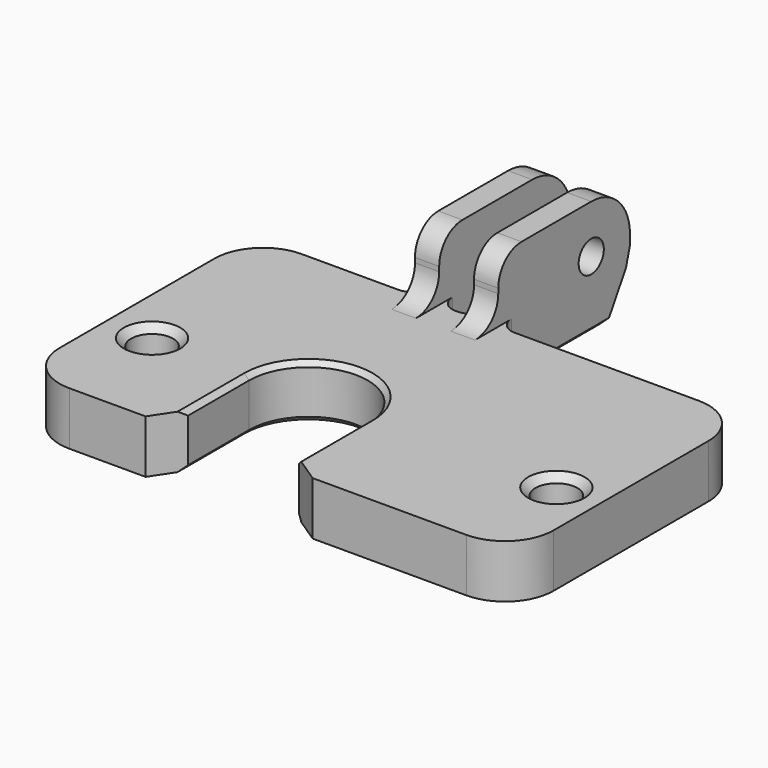
from build123d import *

# Parameters (mm, degrees)
F0_R          = 2.1666665
F1_DEPTH      = 5.5
F2_SIZE       = 0.75
F3_W          = 51
F3_H          = 8
F4_DEPTH      = 5.5
F5_SIZE       = 0.5
F6_W          = 2.5
F6_H          = 17
F7_DEPTH      = 12
F8_R          = 1.625
F9_DEPTH      = 25.301
F10_T1_DEPTH  = 2.5
F10_T3_DEPTH  = 2.5
F10_T8_DEPTH  = 17.5
F10_T14_DEPTH = 17.5
F10_T17_DEPTH = 17.5
F10_T19_DEPTH = 17.5
F11_R         = 5
F12_SIZE2     = 3
F12_SIZE      = 5
F12_2_SIZE2   = 3
F12_2_SIZE    = 5
F13_SIZE      = 1
F14_R         = 5
F15_SIZE2     = 2
F15_SIZE      = 3
F15_2_SIZE2   = 2
F15_2_SIZE    = 3
F16_T1_DEPTH  = 15.285841494
F16_T3_DEPTH  = 4.0033035506
F16_T5_DEPTH  = 4.0033035506
F17_R         = 1.7


# Not quite as in the source:
# - a fillet or chamfer that OpenCascade refuses, or shapes differently, is made with other operations: its cross-section is extruded or revolved along the edge and cut away or added


with BuildPart() as f1:
    # F0 (on Top) → F1 (new body)
    with BuildSketch(Plane.XY):
        with BuildLine():
            Line((25.5, 11), (-25.5, 11))
            Line((-25.5, 11), (-25.5, -11))
            Line((-25.5, -11), (-10.625, -11))
            Line((-10.625, -11), (-10.625, -0.125))
            ThreePointArc((-10.625, -0.125), (-4.5, 6), (1.625, -0.125))
            Line((1.625, -0.125), (1.625, -11))
            Line((1.625, -11), (25.5, -11))
            Line((25.5, -11), (25.5, 11))
        make_face()
        with Locations((-20.75, 0)):
            Circle(F0_R, mode=Mode.SUBTRACT)
        with Locations((21, 0)):
            Circle(F0_R, mode=Mode.SUBTRACT)
    extrude(amount=F1_DEPTH)

    # F2
    f2_edges = [f1.edges().sort_by_distance(p)[0] for p in [
        (-22.916666, 0, 0),
        (18.833334, 0, 0),
        (18.833334, 0, 5.5),
        (-22.916666, 0, 5.5),
    ]]
    chamfer(f2_edges, length=F2_SIZE)

    # F3 (on Top) → F4 (join, through all)
    with BuildSketch(Plane.XY):
        with Locations((0, 15)):
            Rectangle(F3_W, F3_H)
    extrude(amount=F4_DEPTH)

    # F5
    f5_edges = [f1.edges().sort_by_distance(p)[0] for p in [
        (-4.5, 6, 5.5),
        (-4.5, 6, 0),
        (-10.625, -5.5625, 5.5),
        (-10.625, -5.5625, 0),
        (1.625, -5.5625, 0),
        (1.625, -5.5625, 5.5),
    ]]
    chamfer(f5_edges, length=F5_SIZE)

    # F6 (on Top) → F7 (join)
    with BuildSketch(Plane.XY):
        with Locations((-7.55, 27.5)):
            Rectangle(F6_W, F6_H)
        with Locations((-1.45, 27.5)):
            Rectangle(F6_W, F6_H)
    extrude(amount=F7_DEPTH)

    # F8 (on face) → F9 (cut, through all)
    with BuildSketch(Plane.YZ.offset(-0.2)):
        with Locations((31, 7)):
            Circle(F8_R)
    extrude(amount=-F9_DEPTH, mode=Mode.SUBTRACT)

    # F10: fillet of radius 3 on 5 edges, made by hand

    # F10_s2 → F10_t1 (join)
    with BuildSketch(Plane.YZ.offset(-2.7)):
        with BuildLine():
            ThreePointArc((16, 5.5), (18.1213203436, 6.3786796564), (19, 8.5))
            Line((19, 8.5), (19, 5.5))
            Line((19, 5.5), (16, 5.5))
        make_face()
    extrude(amount=F10_T1_DEPTH)

    # F10_s4 → F10_t3 (join)
    with BuildSketch(Plane.YZ.offset(-8.8)):
        with BuildLine():
            ThreePointArc((16, 5.5), (18.1213203436, 6.3786796564), (19, 8.5))
            Line((19, 8.5), (19, 5.5))
            Line((19, 5.5), (16, 5.5))
        make_face()
    extrude(amount=F10_T3_DEPTH)


with BuildPart() as f10_tool6:
    # F10_s7 → F10_t8 (new body)
    with BuildSketch(Plane.YZ.offset(7.3)):
        with BuildLine():
            ThreePointArc((16, 5.5), (18.1213203436, 6.3786796564), (19, 8.5))
            Line((19, 8.5), (19, 5.5))
            Line((19, 5.5), (16, 5.5))
        make_face()
    extrude(amount=-F10_T8_DEPTH)

    split(bisect_by=Plane.YZ.offset(-6.3), keep=Keep.BOTTOM)

    split(bisect_by=Plane.YZ.offset(-8.8), keep=Keep.TOP)


with BuildPart() as f1_1:
    add(f1.part)

    # F10_t5: union F10_tool6
    add(f10_tool6.part)


with BuildPart() as f10_tool12:
    # F10_s13 → F10_t14 (new body)
    with BuildSketch(Plane.YZ.offset(1.2)):
        with BuildLine():
            ThreePointArc((16, 5.5), (18.1213203436, 6.3786796564), (19, 8.5))
            Line((19, 8.5), (19, 5.5))
            Line((19, 5.5), (16, 5.5))
        make_face()
    extrude(amount=-F10_T14_DEPTH)

    split(bisect_by=Plane.YZ.offset(-0.2), keep=Keep.BOTTOM)

    split(bisect_by=Plane.YZ.offset(-2.7), keep=Keep.TOP)


with BuildPart() as f1_2:
    add(f1_1.part)

    # F10_t11: union F10_tool12
    add(f10_tool12.part)

    # F10_s18 → F10_t17 (cut)
    with BuildSketch(Plane.YZ.offset(-10.2)):
        with BuildLine():
            ThreePointArc((19, 9), (19.8786796564, 11.1213203436), (22, 12))
            Line((22, 12), (19, 12))
            Line((19, 12), (19, 9))
        make_face()
    extrude(amount=F10_T17_DEPTH, mode=Mode.SUBTRACT)

    # F10_s20 → F10_t19 (cut)
    with BuildSketch(Plane.YZ.offset(-16.3)):
        with BuildLine():
            ThreePointArc((19, 9), (19.8786796564, 11.1213203436), (22, 12))
            Line((22, 12), (19, 12))
            Line((19, 12), (19, 9))
        make_face()
    extrude(amount=F10_T19_DEPTH, mode=Mode.SUBTRACT)

    # F11
    f11_edges = [f1_2.edges().sort_by_distance(p)[0] for p in [
        (-1.45, 36, 12),
        (-7.55, 36, 12),
    ]]
    fillet(f11_edges, radius=F11_R)

    # F12
    f12_edges = [f1_2.edges().sort_by_distance(p)[0] for p in [
        (-1.45, 36, 0),
    ]]
    f12_side = f1_2.faces().sort_by_distance((-1.45, 36, 3.5))[0]
    chamfer(f12_edges, length=F12_SIZE, length2=F12_SIZE2, reference=f12_side)

    # F12#2
    f12_2_edges = [f1_2.edges().sort_by_distance(p)[0] for p in [
        (-7.55, 36, 0),
    ]]
    f12_2_side = f1_2.faces().sort_by_distance((-7.55, 36, 3.5))[0]
    chamfer(f12_2_edges, length=F12_2_SIZE, length2=F12_2_SIZE2, reference=f12_2_side)

    # F13
    f13_edges = [f1_2.edges().sort_by_distance(p)[0] for p in [
        (-1.45, 36, 5),
        (-7.55, 36, 5),
    ]]
    chamfer(f13_edges, length=F13_SIZE)

    # F14
    f14_edges = [f1_2.edges().sort_by_distance(p)[0] for p in [
        (25.5, -11, 2.75),
        (-25.5, -11, 2.75),
        (25.5, 19, 2.75),
        (-25.5, 19, 2.75),
    ]]
    fillet(f14_edges, radius=F14_R)

    # F15
    f15_edges = [f1_2.edges().sort_by_distance(p)[0] for p in [
        (-10.625, -11, 2.75),
    ]]
    f15_side = f1_2.faces().sort_by_distance((-10.625, -5.5625, 2.75))[0]
    chamfer(f15_edges, length=F15_SIZE, length2=F15_SIZE2, reference=f15_side)

    # F15#2
    f15_2_edges = [f1_2.edges().sort_by_distance(p)[0] for p in [
        (1.625, -11, 2.75),
    ]]
    f15_2_side = f1_2.faces().sort_by_distance((11.08488, -11, 2.75))[0]
    chamfer(f15_2_edges, length=F15_2_SIZE, length2=F15_2_SIZE2, reference=f15_2_side)

    # F16: chamfer of 0.5 on 6 edges, made by hand

    # F16_s2 → F16_t1 (cut)
    with BuildSketch(Plane.XZ.offset(-34.285841494)):
        Polygon((-0.7, 0), (-0.2, 0.5), (-0.2, 0), align=None)
        Polygon((-2.2, 0), (-2.7, 0.5), (-2.7, 0), align=None)
        Polygon((-6.8, 0), (-6.3, 0.5), (-6.3, 0), align=None)
        Polygon((-8.3, 0), (-8.8, 0.5), (-8.8, 0), align=None)
    extrude(amount=F16_T1_DEPTH, mode=Mode.SUBTRACT)

    # F16_s4 → F16_t3 (cut)
    with BuildSketch(Plane.YZ.offset(-3.4516517753)):
        Polygon((32.7169048105, 0), (33.1456512734, 0.2427521223), (33, 0), align=None)
    extrude(amount=F16_T3_DEPTH, mode=Mode.SUBTRACT)

    # F16_s6 → F16_t5 (cut)
    with BuildSketch(Plane.YZ.offset(-9.5516517753)):
        Polygon((32.7169048105, 0), (33.1456512734, 0.2427521223), (33, 0), align=None)
    extrude(amount=F16_T5_DEPTH, mode=Mode.SUBTRACT)

    # F17
    f17_edges = [f1_2.edges().sort_by_distance(p)[0] for p in [
        (-8.8, 19, 3),
        (-6.3, 19, 3),
        (-2.7, 19, 3),
        (-0.2, 19, 3),
    ]]
    fillet(f17_edges, radius=F17_R)


solid = f1_2.part
